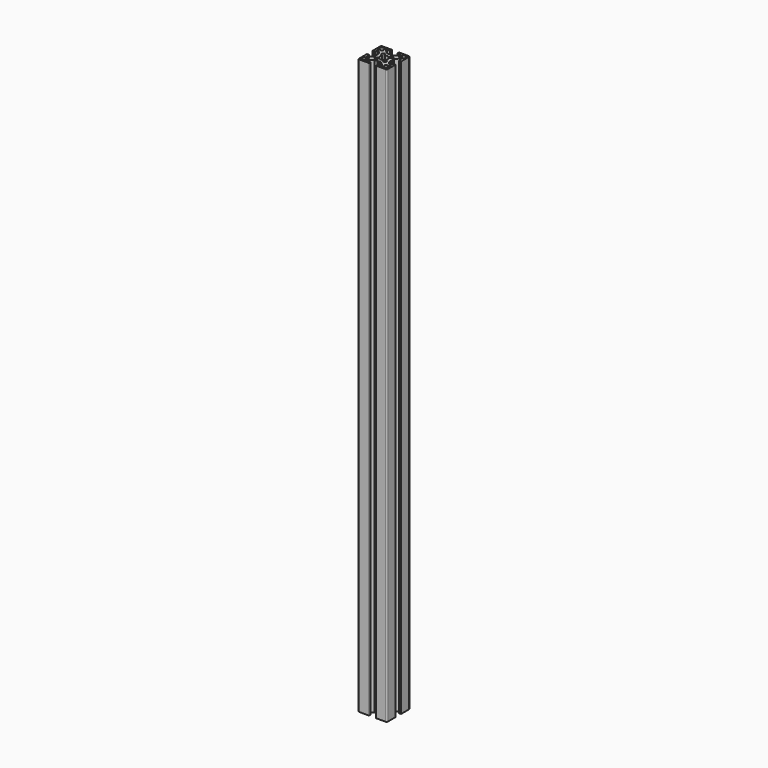
from build123d import *

# Parameters (mm, degrees)
F1_DEPTH = 400


# Not quite as in the source:
# - ends of sketch curves that miss each other by under 0.0002 mm in the source are joined


with BuildPart() as f1:
    # F0 (on Top) → F1 (new body)
    with BuildSketch(Plane.XY):
        with BuildLine():
            ThreePointArc((-769.8592226, 199.4197364), (-770.0935371751, 199.9854218249), (-770.6592226, 200.2197364))
            Line((-770.6592226, 200.2197364), (-777.2192226, 200.2197364))
            ThreePointArc((-777.2192226, 200.2197364), (-777.3889282275, 200.1494420275), (-777.4592226, 199.9797364))
            Line((-777.4592226, 199.9797364), (-777.4592226, 198.8597364))
            ThreePointArc((-777.4592226, 198.8597364), (-777.3889282275, 198.6900307725), (-777.2192226, 198.6197364))
            Line((-777.2192226, 198.6197364), (-775.0592226, 198.6197364))
            Line((-775.0592226, 198.6197364), (-775.0592226, 197.8682644))
            Line((-775.0592226, 197.8682644), (-777.5077506, 195.4197364))
            Line((-777.5077506, 195.4197364), (-779.3363506, 195.4197364))
            ThreePointArc((-779.3363506, 195.4197364), (-779.4398783536, 195.4061066942), (-779.5363508431, 195.3661464211))
            Line((-779.5363508431, 195.3661464211), (-779.8592226, 195.1797364))
            Line((-779.8592226, 195.1797364), (-780.1820938, 195.366146))
            ThreePointArc((-780.1820938, 195.366146), (-780.3820938, 195.4197364), (-780.5820940431, 195.3661464211))
            Line((-780.5820940431, 195.3661464211), (-780.8343306, 195.2205172))
            Line((-780.8343306, 195.2205172), (-781.8592226, 195.4197364))
            Line((-781.8592226, 195.4197364), (-782.2106938, 195.4197364))
            Line((-782.2106938, 195.4197364), (-784.6592226, 197.8682644))
            Line((-784.6592226, 197.8682644), (-784.6592226, 198.6197364))
            Line((-784.6592226, 198.6197364), (-782.4992226, 198.6197364))
            ThreePointArc((-782.4992226, 198.6197364), (-782.3295169725, 198.6900307725), (-782.2592226, 198.8597364))
            Line((-782.2592226, 198.8597364), (-782.2592226, 199.9797364))
            ThreePointArc((-782.2592226, 199.9797364), (-782.3295169725, 200.1494420275), (-782.4992226, 200.2197364))
            Line((-782.4992226, 200.2197364), (-789.0592226, 200.2197364))
            ThreePointArc((-789.0592226, 200.2197364), (-789.6249080249, 199.9854218249), (-789.8592226, 199.4197364))
            Line((-789.8592226, 199.4197364), (-789.8592226, 192.8597364))
            ThreePointArc((-789.8592226, 192.8597364), (-789.7889282275, 192.6900307725), (-789.6192226, 192.6197364))
            Line((-789.6192226, 192.6197364), (-788.4992226, 192.6197364))
            ThreePointArc((-788.4992226, 192.6197364), (-788.3295169725, 192.6900307725), (-788.2592226, 192.8597364))
            Line((-788.2592226, 192.8597364), (-788.2592226, 195.0197364))
            Line((-788.2592226, 195.0197364), (-787.5077506, 195.0197364))
            Line((-787.5077506, 195.0197364), (-785.0592226, 192.5712076))
            Line((-785.0592226, 192.5712076), (-785.0592226, 190.7426076))
            ThreePointArc((-785.0592226, 190.7426076), (-785.0455928942, 190.6390798464), (-785.0056326211, 190.5426073569))
            Line((-785.0056326211, 190.5426073569), (-784.8192226, 190.2197364))
            Line((-784.8192226, 190.2197364), (-785.0056322, 189.8968644))
            ThreePointArc((-785.0056322, 189.8968644), (-785.0592226, 189.6968644), (-785.0056326211, 189.4968641569))
            Line((-785.0056326211, 189.4968641569), (-784.8600034, 189.2446276))
            Line((-784.8600034, 189.2446276), (-785.0592226, 188.2197364))
            Line((-785.0592226, 188.2197364), (-785.0592226, 187.8682644))
            Line((-785.0592226, 187.8682644), (-787.5077506, 185.4197364))
            Line((-787.5077506, 185.4197364), (-788.2592226, 185.4197364))
            Line((-788.2592226, 185.4197364), (-788.2592226, 187.5797364))
            ThreePointArc((-788.2592226, 187.5797364), (-788.3295169725, 187.7494420275), (-788.4992226, 187.8197364))
            Line((-788.4992226, 187.8197364), (-789.6192226, 187.8197364))
            ThreePointArc((-789.6192226, 187.8197364), (-789.7889282275, 187.7494420275), (-789.8592226, 187.5797364))
            Line((-789.8592226, 187.5797364), (-789.8592226, 181.0197364))
            ThreePointArc((-789.8592226, 181.0197364), (-789.6249080249, 180.4540509751), (-789.0592226, 180.2197364))
            Line((-789.0592226, 180.2197364), (-782.4992226, 180.2197364))
            ThreePointArc((-782.4992226, 180.2197364), (-782.3295169725, 180.2900307725), (-782.2592226, 180.4597364))
            Line((-782.2592226, 180.4597364), (-782.2592226, 181.5797364))
            ThreePointArc((-782.2592226, 181.5797364), (-782.3295169725, 181.7494420275), (-782.4992226, 181.8197364))
            Line((-782.4992226, 181.8197364), (-784.6592226, 181.8197364))
            Line((-784.6592226, 181.8197364), (-784.6592226, 182.5712076))
            Line((-784.6592226, 182.5712076), (-782.2106938, 185.0197364))
            Line((-782.2106938, 185.0197364), (-780.3820938, 185.0197364))
            ThreePointArc((-780.3820938, 185.0197364), (-780.2785662395, 185.0333660541), (-780.1820939033, 185.0733261789))
            Line((-780.1820939033, 185.0733261789), (-779.8592226, 185.2597364))
            Line((-779.8592226, 185.2597364), (-779.5363506, 185.073326))
            ThreePointArc((-779.5363506, 185.073326), (-779.3363506, 185.0197364), (-779.1363507033, 185.0733261789))
            Line((-779.1363507033, 185.0733261789), (-778.8841138, 185.2189548))
            Line((-778.8841138, 185.2189548), (-777.8592226, 185.0197364))
            Line((-777.8592226, 185.0197364), (-777.5077506, 185.0197364))
            Line((-777.5077506, 185.0197364), (-775.0592226, 182.5712076))
            Line((-775.0592226, 182.5712076), (-775.0592226, 181.8197364))
            Line((-775.0592226, 181.8197364), (-777.2192226, 181.8197364))
            ThreePointArc((-777.2192226, 181.8197364), (-777.3889282275, 181.7494420275), (-777.4592226, 181.5797364))
            Line((-777.4592226, 181.5797364), (-777.4592226, 180.4597364))
            ThreePointArc((-777.4592226, 180.4597364), (-777.3889282275, 180.2900307725), (-777.2192226, 180.2197364))
            Line((-777.2192226, 180.2197364), (-770.6592226, 180.2197364))
            ThreePointArc((-770.6592226, 180.2197364), (-770.0935371751, 180.4540509751), (-769.8592226, 181.0197364))
            Line((-769.8592226, 181.0197364), (-769.8592226, 187.5797364))
            ThreePointArc((-769.8592226, 187.5797364), (-769.9295169725, 187.7494420275), (-770.0992226, 187.8197364))
            Line((-770.0992226, 187.8197364), (-771.2192226, 187.8197364))
            ThreePointArc((-771.2192226, 187.8197364), (-771.3889282275, 187.7494420275), (-771.4592226, 187.5797364))
            Line((-771.4592226, 187.5797364), (-771.4592226, 185.4197364))
            Line((-771.4592226, 185.4197364), (-772.2106938, 185.4197364))
            Line((-772.2106938, 185.4197364), (-774.6592226, 187.8682644))
            Line((-774.6592226, 187.8682644), (-774.6592226, 189.6968644))
            ThreePointArc((-774.6592226, 189.6968644), (-774.6728522541, 189.8003919605), (-774.7128123789, 189.8968642967))
            Line((-774.7128123789, 189.8968642967), (-774.8992226, 190.2197364))
            Line((-774.8992226, 190.2197364), (-774.7128122, 190.5426076))
            ThreePointArc((-774.7128122, 190.5426076), (-774.6592226, 190.7426076), (-774.7128123789, 190.9426074967))
            Line((-774.7128123789, 190.9426074967), (-774.858441, 191.1948444))
            Line((-774.858441, 191.1948444), (-774.6592226, 192.2197364))
            Line((-774.6592226, 192.2197364), (-774.6592226, 192.5712076))
            Line((-774.6592226, 192.5712076), (-772.2106938, 195.0197364))
            Line((-772.2106938, 195.0197364), (-771.4592226, 195.0197364))
            Line((-771.4592226, 195.0197364), (-771.4592226, 192.8597364))
            ThreePointArc((-771.4592226, 192.8597364), (-771.3889282275, 192.6900307725), (-771.2192226, 192.6197364))
            Line((-771.2192226, 192.6197364), (-770.0992226, 192.6197364))
            ThreePointArc((-770.0992226, 192.6197364), (-769.9295169725, 192.6900307725), (-769.8592226, 192.8597364))
            Line((-769.8592226, 192.8597364), (-769.8592226, 199.4197364))
        make_face()
        with BuildLine():
            Line((-786.3080362, 182.6395516), (-785.8442002, 182.1757156))
            ThreePointArc((-785.8442002, 182.1757156), (-785.72280777, 181.5654334166), (-786.2401802, 181.2197364))
            Line((-786.2401802, 181.2197364), (-787.6592226, 181.2197364))
            ThreePointArc((-787.6592226, 181.2197364), (-788.5077507374, 181.5712082626), (-788.8592226, 182.4197364))
            Line((-788.8592226, 182.4197364), (-788.8592226, 183.838778))
            ThreePointArc((-788.8592226, 183.838778), (-788.5135253221, 184.3561505382), (-787.9032428025, 184.2347577975))
            Line((-787.9032428025, 184.2347577975), (-787.4394066, 183.770922))
            Line((-787.4394066, 183.770922), (-786.8737218, 184.3366076))
            ThreePointArc((-786.8737218, 184.3366076), (-785.7423507751, 184.3366074249), (-785.7423507751, 183.2052365751))
            Line((-785.7423507751, 183.2052365751), (-786.3080362, 182.6395516))
        make_face(mode=Mode.SUBTRACT)
        with BuildLine():
            ThreePointArc((-773.4782642, 181.2197364), (-773.99563663, 181.5654334166), (-773.8742443975, 182.1757157975))
            Line((-773.8742443975, 182.1757157975), (-773.4104082, 182.6395516))
            Line((-773.4104082, 182.6395516), (-773.9760938, 183.2052364))
            ThreePointArc((-773.9760938, 183.2052364), (-773.9760936249, 184.3366074249), (-772.8447227751, 184.3366074249))
            Line((-772.8447227751, 184.3366074249), (-772.2790378, 183.770922))
            Line((-772.2790378, 183.770922), (-771.8152018, 184.234758))
            ThreePointArc((-771.8152018, 184.234758), (-771.2049196166, 184.35615043), (-770.8592226, 183.838778))
            Line((-770.8592226, 183.838778), (-770.8592226, 182.4197364))
            ThreePointArc((-770.8592226, 182.4197364), (-771.2106944626, 181.5712082626), (-772.0592226, 181.2197364))
            Line((-772.0592226, 181.2197364), (-773.4782642, 181.2197364))
        make_face(mode=Mode.SUBTRACT)
        with BuildLine():
            ThreePointArc((-781.0895018686, 192.6455997352), (-779.8592222433, 192.9397364), (-778.6289426951, 192.6455994125))
            ThreePointArc((-778.6289426951, 192.6455994125), (-778.4826210004, 192.6226363415), (-778.3506833725, 192.6899403725))
            Line((-778.3506833725, 192.6899403725), (-777.9549074, 193.0857156))
            ThreePointArc((-777.9549074, 193.0857156), (-776.1822667476, 193.8966914524), (-776.9932426072, 192.1240507016))
            Line((-776.9932426072, 192.1240507016), (-777.3890178, 191.7282748))
            ThreePointArc((-777.3890178, 191.7282748), (-777.4563218585, 191.5963371996), (-777.433359073, 191.4500153601))
            ThreePointArc((-777.433359073, 191.4500153601), (-777.2137785241, 190.8522122031), (-777.1392226, 190.2197364))
            ThreePointArc((-777.1392226, 190.2197364), (-777.2137786071, 189.58726025), (-777.4333594238, 188.9894568178))
            ThreePointArc((-777.4333594238, 188.9894568178), (-777.4563218585, 188.8431348004), (-777.3890178275, 188.7111971725))
            Line((-777.3890178275, 188.7111971725), (-776.9932426, 188.3154212))
            ThreePointArc((-776.9932426, 188.3154212), (-776.1822667476, 186.5427805476), (-777.9549074984, 187.3537564072))
            Line((-777.9549074984, 187.3537564072), (-778.3506834, 187.7495316))
            ThreePointArc((-778.3506834, 187.7495316), (-778.4826208217, 187.81683563), (-778.6289425172, 187.7938730367))
            ThreePointArc((-778.6289425172, 187.7938730367), (-779.8592222433, 187.4997364), (-781.0895018686, 187.7938730648))
            ThreePointArc((-781.0895018686, 187.7938730648), (-781.2358235783, 187.81683563), (-781.3677610275, 187.7495316275))
            Line((-781.3677610275, 187.7495316275), (-781.763537, 187.3537564))
            ThreePointArc((-781.763537, 187.3537564), (-783.5361776524, 186.5427805476), (-782.7252017928, 188.3154212984))
            Line((-782.7252017928, 188.3154212984), (-782.3294266, 188.7111972))
            ThreePointArc((-782.3294266, 188.7111972), (-782.2621225415, 188.8431348004), (-782.285085327, 188.9894566399))
            ThreePointArc((-782.285085327, 188.9894566399), (-782.5792226, 190.2197360433), (-782.2850859352, 191.4500156686))
            ThreePointArc((-782.2850859352, 191.4500156686), (-782.2621225415, 191.5963371996), (-782.3294265725, 191.7282748275))
            Line((-782.3294265725, 191.7282748275), (-782.7252018, 192.1240508))
            ThreePointArc((-782.7252018, 192.1240508), (-783.5361776524, 193.8966914524), (-781.7635369016, 193.0857155928))
            Line((-781.7635369016, 193.0857155928), (-781.367761, 192.6899404))
            ThreePointArc((-781.367761, 192.6899404), (-781.2358233996, 192.6226363415), (-781.0895018686, 192.6455997352))
        make_face(mode=Mode.SUBTRACT)
        with BuildLine():
            ThreePointArc((-786.2401802, 199.2197364), (-785.7228076618, 198.8740391221), (-785.8442004025, 198.2637566025))
            Line((-785.8442004025, 198.2637566025), (-786.3080362, 197.7999204))
            Line((-786.3080362, 197.7999204), (-785.7423506, 197.2342356))
            ThreePointArc((-785.7423506, 197.2342356), (-785.7423507751, 196.1028645751), (-786.8737216249, 196.1028645751))
            Line((-786.8737216249, 196.1028645751), (-787.4394066, 196.66855))
            Line((-787.4394066, 196.66855), (-787.9032426, 196.204714))
            ThreePointArc((-787.9032426, 196.204714), (-788.5135253221, 196.0833214618), (-788.8592226, 196.600694))
            Line((-788.8592226, 196.600694), (-788.8592226, 198.0197364))
            ThreePointArc((-788.8592226, 198.0197364), (-788.5077507374, 198.8682645374), (-787.6592226, 199.2197364))
            Line((-787.6592226, 199.2197364), (-786.2401802, 199.2197364))
        make_face(mode=Mode.SUBTRACT)
        with BuildLine():
            Line((-773.4104082, 197.7999204), (-773.8742442, 198.2637564))
            ThreePointArc((-773.8742442, 198.2637564), (-773.9956367382, 198.8740391221), (-773.4782642, 199.2197364))
            Line((-773.4782642, 199.2197364), (-772.0592226, 199.2197364))
            ThreePointArc((-772.0592226, 199.2197364), (-771.2106944626, 198.8682645374), (-770.8592226, 198.0197364))
            Line((-770.8592226, 198.0197364), (-770.8592226, 196.600694))
            ThreePointArc((-770.8592226, 196.600694), (-771.2049196166, 196.08332157), (-771.8152019975, 196.2047138025))
            Line((-771.8152019975, 196.2047138025), (-772.2790378, 196.66855))
            Line((-772.2790378, 196.66855), (-772.8447226, 196.1028644))
            ThreePointArc((-772.8447226, 196.1028644), (-773.9760936249, 196.1028645751), (-773.9760936249, 197.2342354249))
            Line((-773.9760936249, 197.2342354249), (-773.4104082, 197.7999204))
        make_face(mode=Mode.SUBTRACT)
    extrude(amount=F1_DEPTH)


with BuildPart() as f1_1:
    # F2: moved
    add(f1.part.moved(Location((780.96789, -188.53931, -211.27015))))


solid = f1_1.part
